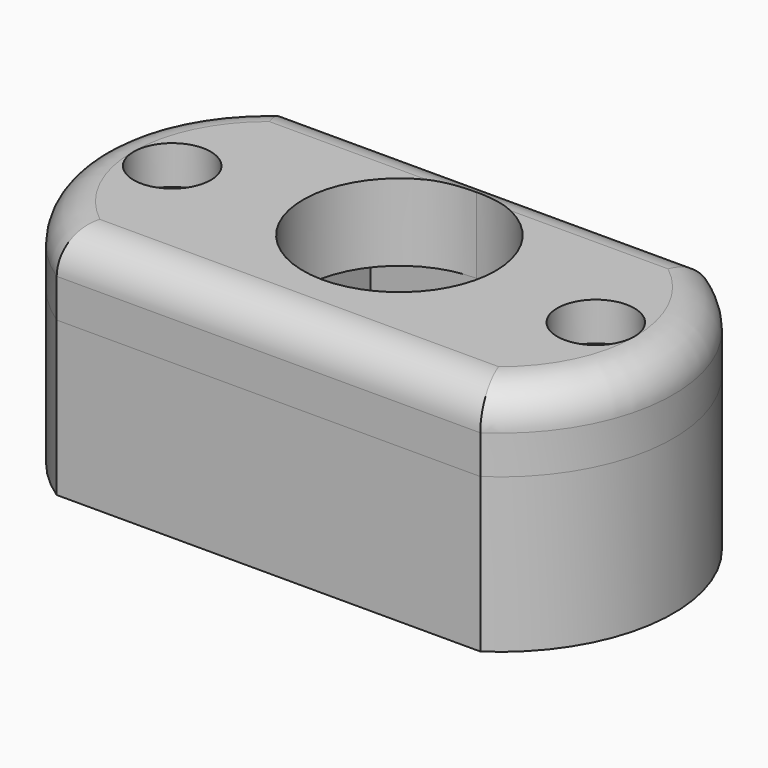
from build123d import *

# Parameters (mm, degrees)
F0_W            = 22
F0_H            = 15
F1_DEPTH        = 8
F2_R            = 1
F2_W            = 11
F2_H            = 12
F3_DEPTH        = 9
F4_W            = 11
F4_H            = 9
F5_DEPTH        = 0.5
F6_W            = 22
F6_H            = 15
F7_DEPTH        = 4
F9_DEPTH        = 4
F10_T1_DEPTH    = 32
F10_T4_ANGLE    = 176.5875970816
F10_T6_ANGLE    = 176.5875970816
F11_D           = 2
F11_DEPTH       = 20
F11_CBORE_D     = 4
F11_CBORE_DEPTH = 2
F11_TIP         = 0.600860619


# Not quite as in the source:
# - a fillet or chamfer that OpenCascade refuses, or shapes differently, is made with other operations: its cross-section is extruded or revolved along the edge and cut away or added


with BuildPart() as f1:
    # F0 (on Top) → F1 (new body)
    with BuildSketch(Plane.XY):
        with Locations((-45, -43.5413755476)):
            Rectangle(F0_W, F0_H)
        with BuildLine():
            ThreePointArc((-34, -51.0413755476), (-29.9749371855, -43.5413755476), (-34, -36.0413755476))
            Line((-34, -36.0413755476), (-34, -51.0413755476))
        make_face()
        with BuildLine():
            Line((-56, -51.0413755476), (-56, -36.0413755476))
            ThreePointArc((-56, -36.0413755476), (-60.0250628145, -43.5413755476), (-56, -51.0413755476))
        make_face()
    extrude(amount=F1_DEPTH)

    # F2 (on face) → F3 (cut)
    with BuildSketch(Plane.XY.offset(8)):
        with Locations((-56, -43.5413755476)):
            Circle(F2_R)
        with Locations((-34, -43.5413755476)):
            Circle(F2_R)
        with Locations((-45, -43.5413755476)):
            Rectangle(F2_W, F2_H)
    extrude(amount=-F3_DEPTH, mode=Mode.SUBTRACT)

    # F4 (on face) → F5 (join)
    with BuildSketch(Plane(origin=(0, 0, 0), x_dir=(1, 0, 0), z_dir=(0, 0, -1))):
        with Locations((-45, 42.0413755476)):
            Rectangle(F4_W, F4_H)
    extrude(amount=-F5_DEPTH)


with BuildPart() as f7:
    # F6 (on face) → F7 (new body)
    with BuildSketch(Plane.XY.offset(8)):
        with Locations((-45, -43.5413755476)):
            Rectangle(F6_W, F6_H)
        with BuildLine():
            ThreePointArc((-34, -51.0413755476), (-29.9749371855, -43.5413755476), (-34, -36.0413755476))
            Line((-34, -36.0413755476), (-34, -51.0413755476))
        make_face()
        with BuildLine():
            Line((-56, -51.0413755476), (-56, -36.0413755476))
            ThreePointArc((-56, -36.0413755476), (-60.0250628145, -43.5413755476), (-56, -51.0413755476))
        make_face()
    extrude(amount=F7_DEPTH)

    # F8 (on face) → F9 (cut)
    with BuildSketch(Plane.XY.offset(12)):
        with BuildLine():
            ThreePointArc((-45, -37.5413755476), (-48.5355339059, -46.0769094536), (-40, -42.5413755476))
            ThreePointArc((-40, -42.5413755476), (-41.4644660941, -39.0058416417), (-45, -37.5413755476))
        make_face()
    extrude(amount=-F9_DEPTH, mode=Mode.SUBTRACT)

    # F10: fillet of radius 2 on 4 edges, made by hand

    # F10_s2 → F10_t1 (cut)
    with BuildSketch(Plane.YZ.offset(-61)):
        with BuildLine():
            ThreePointArc((-36.0413755476, 10), (-36.6271619853, 11.4142135624), (-38.0413755476, 12))
            Line((-38.0413755476, 12), (-36.0413755476, 12))
            Line((-36.0413755476, 12), (-36.0413755476, 10))
        make_face()
        with BuildLine():
            ThreePointArc((-49.0413755476, 12), (-50.45558911, 11.4142135624), (-51.0413755476, 10))
            Line((-51.0413755476, 10), (-51.0413755476, 12))
            Line((-51.0413755476, 12), (-49.0413755476, 12))
        make_face()
    extrude(amount=F10_T1_DEPTH, mode=Mode.SUBTRACT)

    # F10_s3 → F10_t4 (revolve, cut)
    with BuildSketch(Plane(origin=(-40.2362302043, -1.1985422881, 0), x_dir=(0, 0, 1), z_dir=(-0.9995566433, -0.0297744322, 0))):
        with BuildLine():
            ThreePointArc((10, -51.3616145647), (11.4142135624, -50.7758281271), (12, -49.3616145647))
            Line((12, -49.3616145647), (12, -51.3616145647))
            Line((12, -51.3616145647), (10, -51.3616145647))
        make_face()
    revolve(axis=Axis((-38.9749371855, -43.5413755476, 12), (0, 0, 1)), revolution_arc=F10_T4_ANGLE, mode=Mode.SUBTRACT)

    # F10_s5 → F10_t6 (revolve, cut)
    with BuildSketch(Plane(origin=(-52.2756731943, -1.557168866, 0), x_dir=(0, 0, 1), z_dir=(0.9995566433, 0.0297744322, 0))):
        with BuildLine():
            ThreePointArc((10, 33.0028289167), (11.4142135624, 33.5886153543), (12, 35.0028289167))
            Line((12, 35.0028289167), (12, 33.0028289167))
            Line((12, 33.0028289167), (10, 33.0028289167))
        make_face()
    revolve(axis=Axis((-51.0250628145, -43.5413755476, 12), (0, 0, 1)), revolution_arc=F10_T6_ANGLE, mode=Mode.SUBTRACT)

    # F11
    with Locations(Plane.XY.offset(12)):
        with Locations((-34, -43.5413755476), (-56, -43.5413755476)):
            CounterBoreHole(F11_D / 2, F11_CBORE_D / 2, F11_CBORE_DEPTH, depth=F11_DEPTH)
            with Locations((0, 0, -(F11_DEPTH + F11_TIP / 2))):  # 118° drill point
                Cone(0, F11_D / 2, F11_TIP, mode=Mode.SUBTRACT)


solid = Compound([f1.part, f7.part])
